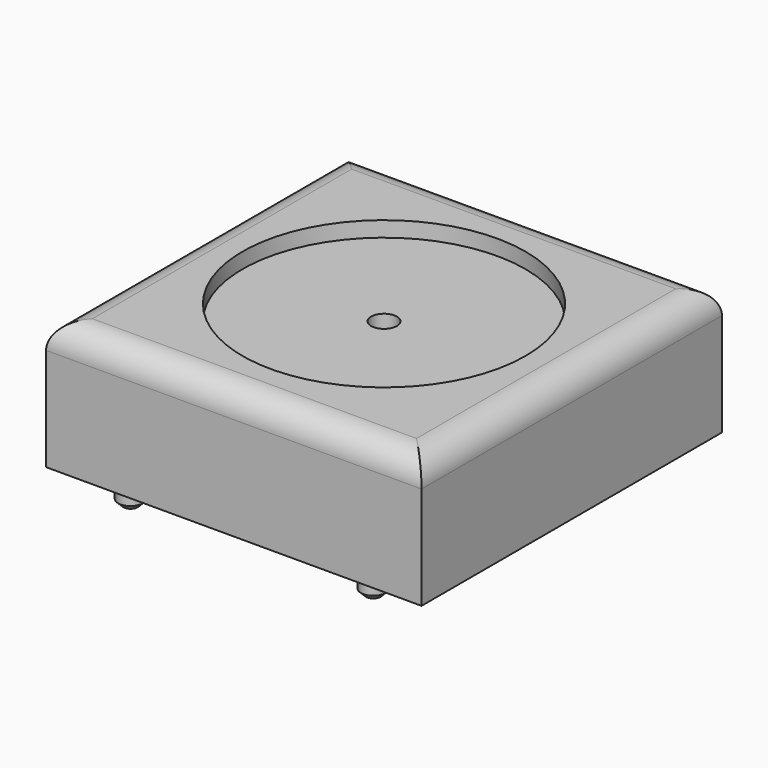
from build123d import *

# Parameters (mm, degrees)
F0_W      = 73
F0_H      = 73
F1_DEPTH  = 25
F2_R      = 5
F3_R      = 27.5
F4_DEPTH  = 3
F5_R      = 2.4
F6_DEPTH  = 4
F7_SIZE   = 1
F9_W      = 110.5126142502
F9_H      = 98.0203673244
F10_DEPTH = 40.1
F14_D     = 5


# Not quite as in the source:
# - a feature of the source that left no trace in its solid (it failed there, or was rolled back) is left out


with BuildPart() as f1:
    # F0 (on Top) → F1 (new body)
    with BuildSketch(Plane.XY):
        Rectangle(F0_W, F0_H)
    extrude(amount=F1_DEPTH)

    # F2
    f2_edges = [f1.edges().sort_by_distance(p)[0] for p in [
        (0, 36.5, 25),
        (0, -36.5, 25),
        (36.5, 0, 25),
        (-36.5, 0, 25),
    ]]
    fillet(f2_edges, radius=F2_R)

    # F3 (on face) → F4 (cut)
    with BuildSketch(Plane.XY.offset(25)):
        Circle(F3_R)
    extrude(amount=-F4_DEPTH, mode=Mode.SUBTRACT)

    # F5 (on face) → F6 (join)
    with BuildSketch(Plane.XY):
        with Locations((-23.6, -32.1)):
            Circle(F5_R)
        with Locations((23.6, -32.1)):
            Circle(F5_R)
        with Locations((-23.6, 32.1)):
            Circle(F5_R)
        with Locations((23.6, 32.1)):
            Circle(F5_R)
    extrude(amount=-F6_DEPTH)

    # F7
    f7_edges = [f1.edges().sort_by_distance(p)[0] for p in [
        (-26, -32.1, -4),
        (-26, 32.1, -4),
        (21.2, 32.1, -4),
        (21.2, -32.1, -4),
    ]]
    chamfer(f7_edges, length=F7_SIZE)

    # F14 (through all)
    with Locations(Plane.XY.offset(22)):
        with Locations((0, 0)):
            Hole(F14_D / 2)


with BuildPart() as f10:
    # F9 (on offset) → F10 (new body, through all)
    with BuildSketch(Plane.XY.offset(40.1)):
        Rectangle(F9_W, F9_H)
    extrude(amount=-F10_DEPTH)


solid = f1.part
